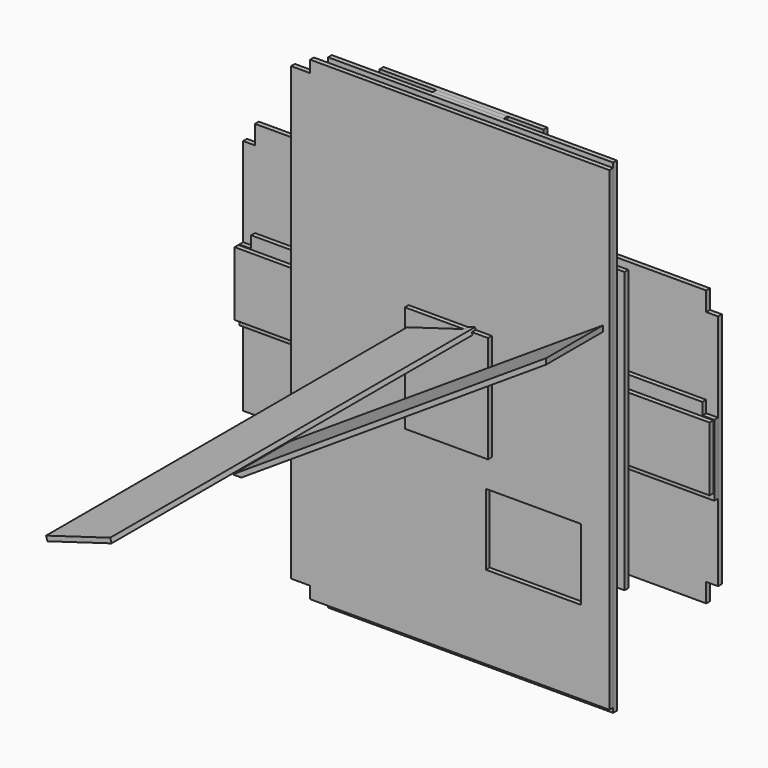
from build123d import *

# Parameters (mm, degrees)
F1_DEPTH  = 20
F3_DEPTH  = 20
F4_W      = 320
F4_H      = 270
F5_DEPTH  = 20
F6_W      = 2000
F6_H      = 270
F7_DEPTH  = 20
F9_DEPTH  = 2040
F10_W     = 1340
F10_H     = 1180
F11_DEPTH = 20
F12_W     = 690
F12_H     = 2040
F13_DEPTH = 20
F14_W     = 300
F14_H     = 2040
F15_DEPTH = 20
F16_W     = 1200
F16_H     = 2040
F17_DEPTH = 20
F18_W     = 0.3014054894
F18_H     = 2000
F18_W_2   = 1200
F19_DEPTH = 20
F20_W     = 400
F20_H     = 300
F21_DEPTH = 25
F22_W     = 350
F22_H     = 450
F23_DEPTH = 20
F25_DEPTH = 300


with BuildPart() as f1:
    # F0 (on Front) → F1 (new body)
    with BuildSketch(Plane.XZ):
        Polygon((950, 500), (950, 580), (-950, 580), (-950, 500), (-1000, 500), (-1000, -500), (-950, -500), (-950, -580), (950, -580), (950, -500), (1000, -500), (1000, 500), align=None)
    extrude(amount=F1_DEPTH)


with BuildPart() as f3:
    # F2 (on face) → F3 (new body)
    with BuildSketch(Plane.XZ.offset(20)):
        Polygon((950, 125), (950, 175), (-950, 175), (-950, 125), (-1000, 125), (-1000, -175), (1000, -175), (1000, 125), align=None)
    extrude(amount=F3_DEPTH)


with BuildPart() as f5:
    # F4 (on face) → F5 (new body)
    with BuildSketch(Plane.XZ.offset(40)):
        Rectangle(F4_W, F4_H)
        Polygon((-160, 135), (160, 135), (160, 215), (110, 215), align=None)
    extrude(amount=F5_DEPTH)


with BuildPart() as f7:
    # F6 (on face) → F7 (new body)
    with BuildSketch(Plane.XZ.offset(60)):
        with Locations((12.1596539393, 0)):
            Rectangle(F6_W, F6_H)
    extrude(amount=F7_DEPTH)


with BuildPart() as f9:
    # F8 (on face) → F9 (new body)
    with BuildSketch(Plane.XZ.offset(60)):
        Polygon((-160, 135), (110, 215), (104.3182334062, 234.1759622542), (-165.6817665938, 154.1759622542), align=None)
    extrude(amount=F9_DEPTH)


with BuildPart() as f11:
    # F10 (on face) → F11 (new body)
    with BuildSketch(Plane.XZ.offset(80)):
        Rectangle(F10_W, F10_H)
    extrude(amount=F11_DEPTH)


with BuildPart() as f13:
    # F12 (on face) → F13 (new body)
    with BuildSketch(Plane.XZ.offset(100)):
        Rectangle(F12_W, F12_H)
    extrude(amount=F13_DEPTH)


with BuildPart() as f15:
    # F14 (on face) → F15 (new body)
    with BuildSketch(Plane.XZ.offset(120)):
        with Locations((43.2888381183, 0)):
            Rectangle(F14_W, F14_H)
    extrude(amount=F15_DEPTH)


with BuildPart() as f17:
    # F16 (on face) → F17 (new body)
    with BuildSketch(Plane.XZ.offset(140)):
        with Locations((69.6985945106, 0)):
            Rectangle(F16_W, F16_H)
    extrude(amount=F17_DEPTH)


with BuildPart() as f19:
    # F18 (on face) → F19 (new body)
    with BuildSketch(Plane.XZ.offset(160)):
        with Locations((669.8492972553, 0)):
            Rectangle(F18_W, F18_H)
        Polygon((-530.3014054894, 1000), (-590, 1000), (-590, 950), (-670, 950), (-670, -950), (-590, -950), (-590, -1000), (-530.3014054894, -1000), align=None)
        with Locations((69.6985945106, 0)):
            Rectangle(F18_W_2, F18_H)
    extrude(amount=F19_DEPTH)

    # F20 (on face) → F21 (cut)
    with BuildSketch(Plane.XZ.offset(180)):
        with Locations((350, -500)):
            Rectangle(F20_W, F20_H)
    extrude(amount=-F21_DEPTH, mode=Mode.SUBTRACT)


with BuildPart() as f23:
    # F22 (on face) → F23 (new body)
    with BuildSketch(Plane.XZ.offset(180)):
        Rectangle(F22_W, F22_H)
    extrude(amount=F23_DEPTH)


with BuildPart() as f25:
    # F24 (on face) → F25 (new body)
    with BuildSketch(Plane.XZ.offset(200)):
        Polygon((660, 430), (-660, -430), (-623.3619430822, -430), (660, 406.129750796), align=None)
    extrude(amount=F25_DEPTH)


solid = Compound([f1.part, f3.part, f5.part, f7.part, f9.part, f11.part, f13.part, f15.part, f17.part, f19.part, f23.part, f25.part])
